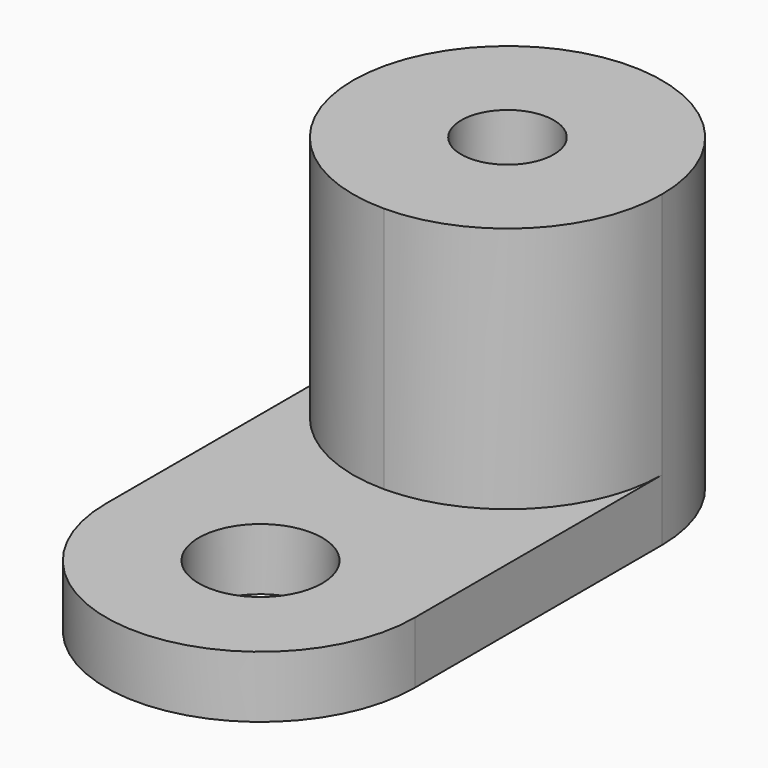
from build123d import *

# Parameters (mm, degrees)
F0_R     = 1.5
F1_DEPTH = 10
F0_R_2   = 2
F2_DEPTH = 2
F3_DEPTH = 5


# Not quite as in the source:
# - a feature names something its author has since deleted; it is built from what else it names


with BuildPart() as f1:
    # F0 (on Top) → F1 (new body)
    with BuildSketch(Plane.XY):
        with BuildLine():
            ThreePointArc((-5, 17.7205532079), (-3.5355338943, 14.1850192903), (3.3e-08, 12.7205532079))
            ThreePointArc((3.3e-08, 12.7205532079), (3.5355339176, 14.1850193136), (5, 17.7205532079))
            ThreePointArc((5, 17.7205532079), (0, 22.7205532079), (-5, 17.7205532079))
        make_face()
        Polygon((-2.8123748533, 16.2461445068), (-2.6830628173, 19.4189369253), (0.129312036, 20.8933456263), (2.8123748533, 19.1949619089), (2.6830628173, 16.0221694904), (-0.129312036, 14.5477607894), align=None, mode=Mode.SUBTRACT)
        Polygon((0.129312036, 20.8933456263), (-2.6830628173, 19.4189369253), (-2.8123748533, 16.2461445068), (-0.129312036, 14.5477607894), (2.6830628173, 16.0221694904), (2.8123748533, 19.1949619089), align=None)
        with Locations((0, 17.7205532079)):
            Circle(F0_R, mode=Mode.SUBTRACT)
    extrude(amount=F1_DEPTH)

    # F0 (on Top) → F2 (join)
    with BuildSketch(Plane.XY):
        with BuildLine():
            ThreePointArc((3.3e-08, 12.7205532079), (3.5355339176, 11.2560871021), (5, 7.7205532079))
            Line((5, 7.7205532079), (5, 17.7205532079))
            ThreePointArc((5, 17.7205532079), (3.5355339176, 14.1850193136), (3.3e-08, 12.7205532079))
        make_face()
        with BuildLine():
            ThreePointArc((3.3e-08, 12.7205532079), (-3.5355338943, 11.2560871255), (-5, 7.7205532079))
            ThreePointArc((-5, 7.7205532079), (0, 2.7205532079), (5, 7.7205532079))
            ThreePointArc((5, 7.7205532079), (3.5355339176, 11.2560871021), (3.3e-08, 12.7205532079))
        make_face()
        with Locations((0, 7.7205532079)):
            Circle(F0_R_2, mode=Mode.SUBTRACT)
        with BuildLine():
            Line((-5, 17.7205532079), (-5, 7.7205532079))
            ThreePointArc((-5, 7.7205532079), (-3.5355338943, 11.2560871255), (3.3e-08, 12.7205532079))
            ThreePointArc((3.3e-08, 12.7205532079), (-3.5355338943, 14.1850192903), (-5, 17.7205532079))
        make_face()
    extrude(amount=F2_DEPTH)

    # F0 (on Top) → F3 (cut)
    with BuildSketch(Plane.XY):
        Polygon((0.129312036, 20.8933456263), (-2.6830628173, 19.4189369253), (-2.8123748533, 16.2461445068), (-0.129312036, 14.5477607894), (2.6830628173, 16.0221694904), (2.8123748533, 19.1949619089), align=None)
        with Locations((0, 17.7205532079)):
            Circle(F0_R, mode=Mode.SUBTRACT)
    extrude(amount=F3_DEPTH, mode=Mode.SUBTRACT)


solid = f1.part
